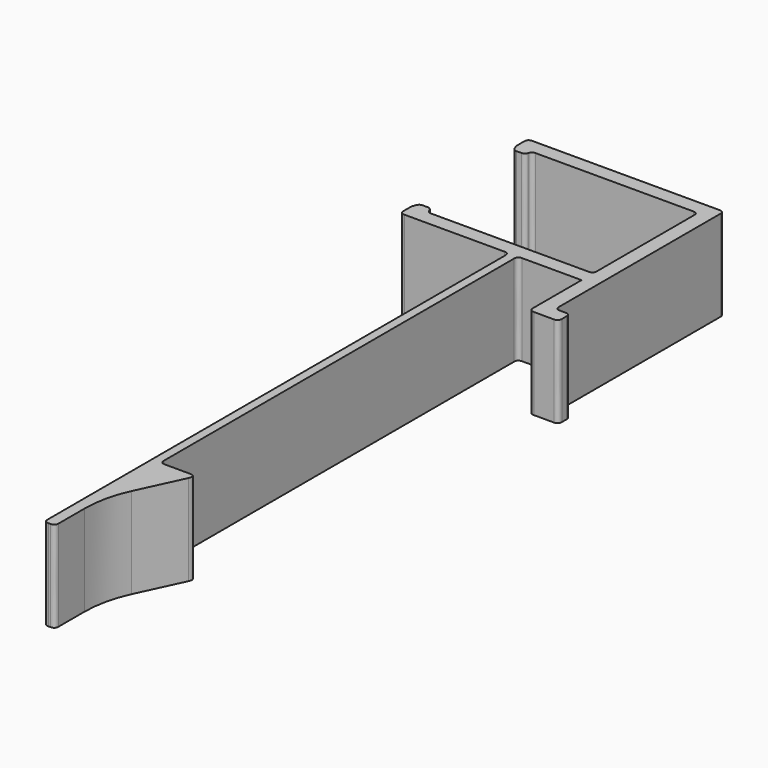
from build123d import *

# Parameters (mm, degrees)
F0_W        = 4
F0_H        = 4
F1_DEPTH    = 25
F2_T1_DEPTH = 25
F2_T3_DEPTH = 31.25
F2_T5_DEPTH = 29.2137491404
F2_T7_DEPTH = 26.2162531519
F2_T9_DEPTH = 34.810534857
F3_R        = 30


# Not quite as in the source:
# - a fillet or chamfer that OpenCascade refuses, or shapes differently, is made with other operations: its cross-section is extruded or revolved along the edge and cut away or added


with BuildPart() as f1:
    # F0 (on Top) → F1 (new body)
    with BuildSketch(Plane.XY):
        Polygon((54, 0), (0, 0), (0, -4), (4.5, -4), (50, -4), (50, -40), (4.5, -40), (0, -40), (0, -44), (30, -44), (30, -204), (33, -204), (33, -187.1583650528), (42.4, -167), (32.4, -167), (32.4, -44), (50, -44), (50, -62), (54, -62), (54, -58), align=None)
        Polygon((4.5, -4), (0, -4), (0.75, -5.8540496218), (3.75, -5.8540496218), align=None)
        with Locations((56, -60)):
            Rectangle(F0_W, F0_H)
        Polygon((0, -40), (4.5, -40), (3.75, -38.1459503782), (0.75, -38.1459503782), align=None)
    extrude(amount=F1_DEPTH)

    # F2: fillet of radius 1.25 on 23 edges, made by hand

    # F2_s2 → F2_t1 (join)
    with BuildSketch(Plane.XY):
        with BuildLine():
            add(Edge.make_bspline(
                [(4.1839688145, -4.78125), (4.5, -4), (5.3427498281, -4)],
                knots=[0, 0, 0, 1, 1, 1], degree=2, weights=[1, 1, 1]))
            Line((5.3427498281, -4), (4.5, -4))
            Line((4.5, -4), (4.1839688145, -4.78125))
        make_face()
        with BuildLine():
            add(Edge.make_bspline(
                [(5.3427498281, -40), (4.5, -40), (4.1839688145, -39.21875)],
                knots=[0, 0, 0, 1, 1, 1], degree=2, weights=[1, 1, 1]))
            Line((4.1839688145, -39.21875), (4.5, -40))
            Line((4.5, -40), (5.3427498281, -40))
        make_face()
        with BuildLine():
            add(Edge.make_bspline(
                [(50, -38.75), (50, -40), (48.75, -40)],
                knots=[0, 0, 0, 1, 1, 1], degree=2, weights=[1, 1, 1]))
            Line((48.75, -40), (50, -40))
            Line((50, -40), (50, -38.75))
        make_face()
        with BuildLine():
            add(Edge.make_bspline(
                [(48.75, -4), (50, -4), (50, -5.25)],
                knots=[0, 0, 0, 1, 1, 1], degree=2, weights=[1, 1, 1]))
            Line((50, -5.25), (50, -4))
            Line((50, -4), (48.75, -4))
        make_face()
        with BuildLine():
            add(Edge.make_bspline(
                [(55.25, -58), (54, -58), (54, -56.75)],
                knots=[0, 0, 0, 1, 1, 1], degree=2, weights=[1, 1, 1]))
            Line((54, -56.75), (54, -58))
            Line((54, -58), (55.25, -58))
        make_face()
        with BuildLine():
            add(Edge.make_bspline(
                [(28.75, -44), (30, -44), (30, -45.25)],
                knots=[0, 0, 0, 1, 1, 1], degree=2, weights=[1, 1, 1]))
            Line((30, -45.25), (30, -44))
            Line((30, -44), (28.75, -44))
        make_face()
        with BuildLine():
            add(Edge.make_bspline(
                [(32.4, -45.25), (32.4, -44), (33.65, -44)],
                knots=[0, 0, 0, 1, 1, 1], degree=2, weights=[1, 1, 1]))
            Line((33.65, -44), (32.4, -44))
            Line((32.4, -44), (32.4, -45.25))
        make_face()
        with BuildLine():
            add(Edge.make_bspline(
                [(33.65, -167), (32.4, -167), (32.4, -165.75)],
                knots=[0, 0, 0, 1, 1, 1], degree=2, weights=[1, 1, 1]))
            Line((32.4, -165.75), (32.4, -167))
            Line((32.4, -167), (33.65, -167))
        make_face()
    extrude(amount=F2_T1_DEPTH)

    # F2_s4 → F2_t3 (cut)
    with BuildSketch(Plane.XY.offset(-3.125)):
        with BuildLine():
            add(Edge.make_bspline(
                [(31.75, -204), (33, -204), (33, -202.75)],
                knots=[0, 0, 0, 1, 1, 1], degree=2, weights=[1, 1, 1]))
            Line((33, -202.75), (33, -204))
            Line((33, -204), (31.75, -204))
        make_face()
        with BuildLine():
            add(Edge.make_bspline(
                [(30, -202.75), (30, -204), (31.25, -204)],
                knots=[0, 0, 0, 1, 1, 1], degree=2, weights=[1, 1, 1]))
            Line((31.25, -204), (30, -204))
            Line((30, -204), (30, -202.75))
        make_face()
        with BuildLine():
            add(Edge.make_bspline(
                [(1.25, 0), (0, 0), (0, -1.25)],
                knots=[0, 0, 0, 1, 1, 1], degree=2, weights=[1, 1, 1]))
            Line((0, -1.25), (0, 0))
            Line((0, 0), (1.25, 0))
        make_face()
        with BuildLine():
            add(Edge.make_bspline(
                [(0, -42.75), (0, -44), (1.25, -44)],
                knots=[0, 0, 0, 1, 1, 1], degree=2, weights=[1, 1, 1]))
            Line((1.25, -44), (0, -44))
            Line((0, -44), (0, -42.75))
        make_face()
        with BuildLine():
            add(Edge.make_bspline(
                [(52.75, 0), (54, 0), (54, -1.25)],
                knots=[0, 0, 0, 1, 1, 1], degree=2, weights=[1, 1, 1]))
            Line((54, -1.25), (54, 0))
            Line((54, 0), (52.75, 0))
        make_face()
        with BuildLine():
            add(Edge.make_bspline(
                [(58, -59.25), (58, -58), (56.75, -58)],
                knots=[0, 0, 0, 1, 1, 1], degree=2, weights=[1, 1, 1]))
            Line((56.75, -58), (58, -58))
            Line((58, -58), (58, -59.25))
        make_face()
        with BuildLine():
            add(Edge.make_bspline(
                [(56.75, -62), (58, -62), (58, -60.75)],
                knots=[0, 0, 0, 1, 1, 1], degree=2, weights=[1, 1, 1]))
            Line((58, -60.75), (58, -62))
            Line((58, -62), (56.75, -62))
        make_face()
        with BuildLine():
            add(Edge.make_bspline(
                [(50, -60.75), (50, -62), (51.25, -62)],
                knots=[0, 0, 0, 1, 1, 1], degree=2, weights=[1, 1, 1]))
            Line((51.25, -62), (50, -62))
            Line((50, -62), (50, -60.75))
        make_face()
    extrude(amount=F2_T3_DEPTH, mode=Mode.SUBTRACT)

    # F2_s6 → F2_t5 (cut)
    with BuildSketch(Plane.XY.offset(-2.1068745702)):
        with BuildLine():
            add(Edge.make_bspline(
                [(2.9072501719, -5.8540496218), (3.75, -5.8540496218), (4.0660311855, -5.0727996218)],
                knots=[0, 0, 0, 1, 1, 1], degree=2, weights=[1, 1, 1]))
            Line((4.0660311855, -5.0727996218), (3.75, -5.8540496218))
            Line((3.75, -5.8540496218), (2.9072501719, -5.8540496218))
        make_face()
        with BuildLine():
            add(Edge.make_bspline(
                [(0.4339688145, -5.0727996218), (0.75, -5.8540496218), (1.5927498281, -5.8540496218)],
                knots=[0, 0, 0, 1, 1, 1], degree=2, weights=[1, 1, 1]))
            Line((1.5927498281, -5.8540496218), (0.75, -5.8540496218))
            Line((0.75, -5.8540496218), (0.4339688145, -5.0727996218))
        make_face()
        with BuildLine():
            add(Edge.make_bspline(
                [(1.5927498281, -38.1459503782), (0.75, -38.1459503782), (0.4339688145, -38.9272003782)],
                knots=[0, 0, 0, 1, 1, 1], degree=2, weights=[1, 1, 1]))
            Line((0.4339688145, -38.9272003782), (0.75, -38.1459503782))
            Line((0.75, -38.1459503782), (1.5927498281, -38.1459503782))
        make_face()
        with BuildLine():
            add(Edge.make_bspline(
                [(4.0660311855, -38.9272003782), (3.75, -38.1459503782), (2.9072501719, -38.1459503782)],
                knots=[0, 0, 0, 1, 1, 1], degree=2, weights=[1, 1, 1]))
            Line((2.9072501719, -38.1459503782), (3.75, -38.1459503782))
            Line((3.75, -38.1459503782), (4.0660311855, -38.9272003782))
        make_face()
    extrude(amount=F2_T5_DEPTH, mode=Mode.SUBTRACT)

    # F2_s8 → F2_t7 (cut)
    with BuildSketch(Plane.XY.offset(-0.6081265759)):
        with BuildLine():
            add(Edge.make_bspline(
                [(0, -3.7567493696), (0, -4), (0.0912189864, -4.2254993696)],
                knots=[0, 0, 0, 1, 1, 1], degree=2, weights=[1, 1, 1]))
            Line((0.0912189864, -4.2254993696), (0, -4))
            Line((0, -4), (0, -3.7567493696))
        make_face()
        with BuildLine():
            add(Edge.make_bspline(
                [(0.0912189864, -39.7745006304), (0, -40), (0, -40.2432506304)],
                knots=[0, 0, 0, 1, 1, 1], degree=2, weights=[1, 1, 1]))
            Line((0, -40.2432506304), (0, -40))
            Line((0, -40), (0.0912189864, -39.7745006304))
        make_face()
    extrude(amount=F2_T7_DEPTH, mode=Mode.SUBTRACT)

    # F2_s10 → F2_t9 (cut)
    with BuildSketch(Plane.XY.offset(-4.9052674285)):
        with BuildLine():
            add(Edge.make_bspline(
                [(41.5707777624, -168.7782728272), (42.4, -167), (40.4378930286, -167)],
                knots=[0, 0, 0, 1, 1, 1], degree=2, weights=[1, 1, 1]))
            Line((40.4378930286, -167), (42.4, -167))
            Line((42.4, -167), (41.5707777624, -168.7782728272))
        make_face()
    extrude(amount=F2_T9_DEPTH, mode=Mode.SUBTRACT)

    # F3
    f3_edges = [f1.edges().sort_by_distance(p)[0] for p in [
        (33, -187.158365, 12.5),
    ]]
    fillet(f3_edges, radius=F3_R)


solid = f1.part
